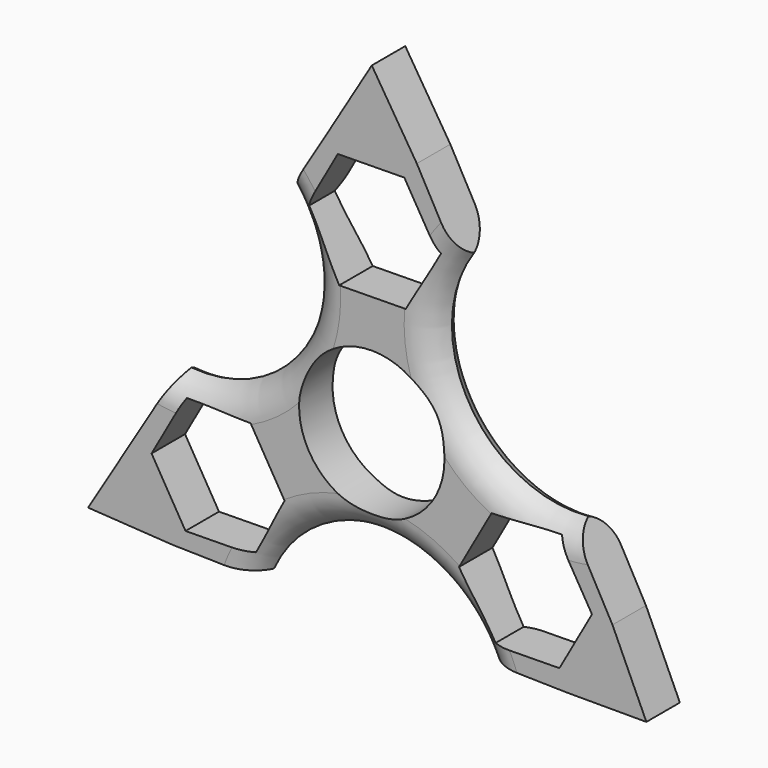
from build123d import *

# Parameters (mm, degrees)
F0_R        = 11.0236
F1_DEPTH    = 6.35
F3_DEPTH    = 6.351
F4_T2_ANGLE = 208.5230453718
F4_T4_ANGLE = 208.5230453718
F5_T2_ANGLE = 208.2569574015
F5_T4_ANGLE = 208.2569574015
F5_T6_ANGLE = 208.3391735822
F5_T8_ANGLE = 208.3391735822


# Not quite as in the source:
# - a fillet or chamfer that OpenCascade refuses, or shapes differently, is made with other operations: its cross-section is extruded or revolved along the edge and cut away or added


with BuildPart() as f1:
    # F0 (on Front) → F1 (new body)
    with BuildSketch(Plane.XZ):
        with BuildLine():
            ThreePointArc((-6.361134185, 38.4869140134), (-13.0376894815, 34.8143114794), (-13.1954000372, 27.1959437158))
            Line((-13.1954000372, 27.1959437158), (-6.361134185, 38.4869140134))
        make_face()
        with BuildLine():
            ThreePointArc((-13.1954000372, 27.1959437158), (-12.0854365863, 25.4236919745), (-11.182896614, 23.5373418757))
            Line((-11.182896614, 23.5373418757), (-6.8342658522, 15.6318107228))
            Line((-6.8342658522, 15.6318107228), (6.361134185, 15.3586480274))
            Line((6.361134185, 15.3586480274), (12.166239176, 24.9493296669))
            ThreePointArc((12.166239176, 24.9493296669), (12.6579537914, 25.813314353), (13.1954000372, 26.649618325))
            Line((13.1954000372, 26.649618325), (6.8342658522, 38.213751318))
            Line((6.8342658522, 38.213751318), (-6.361134185, 38.4869140134))
            Line((-6.361134185, 38.4869140134), (-13.1954000372, 27.1959437158))
        make_face()
        Polygon((-5.1509550469, 35.5981407892), (4.9376044233, 35.7213188292), (10.0885594702, 27.0459590603), (5.1509550469, 18.2474212516), (-4.9376044233, 18.1242432116), (-10.0885594702, 26.7996029805), align=None, mode=Mode.SUBTRACT)
        Polygon((0, 49.0980930626), (-6.361134185, 38.4869140134), (6.8342658522, 38.213751318), align=None)
        with BuildLine():
            ThreePointArc((13.1954000372, 26.649618325), (13.3531105929, 34.2679860885), (6.8342658522, 38.213751318))
            Line((6.8342658522, 38.213751318), (13.1954000372, 26.649618325))
        make_face()
        with BuildLine():
            ThreePointArc((-12.0743322028, 7.6382693135), (3.9762189893, 13.7230586532), (14.2875, 0))
            ThreePointArc((14.2875, 0), (10.1308119649, -10.0746863565), (0.0793732905, -14.2872795217))
            ThreePointArc((0.0793732905, -14.2872795217), (8.9083466238, -16.6700675471), (15.5142475213, -22.9938735391))
            Line((15.5142475213, -22.9938735391), (10.120412267, -13.1882278148))
            Line((10.120412267, -13.1882278148), (16.9546781192, -1.8972575172))
            Line((16.9546781192, -1.8972575172), (26.036317183, -2.0852597754))
            ThreePointArc((26.036317183, -2.0852597754), (12.024896146, 7.8015018829), (12.166239176, 24.9493296669))
            Line((12.166239176, 24.9493296669), (6.361134185, 15.3586480274))
            Line((6.361134185, 15.3586480274), (-6.8342658522, 15.6318107228))
            Line((-6.8342658522, 15.6318107228), (-11.182896614, 23.5373418757))
            ThreePointArc((-11.182896614, 23.5373418757), (-9.8273821058, 15.4868133781), (-12.0743322028, 7.6382693135))
        make_face()
        with BuildLine():
            ThreePointArc((-0.2295262012, -14.2856562318), (-12.3235568651, -7.229287824), (-12.5815056316, 6.7704041454))
            ThreePointArc((-12.5815056316, 6.7704041454), (-19.015460222, 0.5347397877), (-27.6268738812, -1.9396968034))
            Line((-27.6268738812, -1.9396968034), (-16.481546452, -2.1704202126))
            Line((-16.481546452, -2.1704202126), (-10.120412267, -13.7345532056))
            Line((-10.120412267, -13.7345532056), (-14.8142929381, -21.48936819))
            ThreePointArc((-14.8142929381, -21.48936819), (-8.3570392335, -16.196693448), (-0.2295262012, -14.2856562318))
        make_face()
        with BuildLine():
            Line((-16.481546452, -2.1704202126), (-27.6268738812, -1.9396968034))
            ThreePointArc((-27.6268738812, -1.9396968034), (-28.6524995261, -1.9469458697), (-29.6769464892, -1.8972575172))
            Line((-29.6769464892, -1.8972575172), (-36.5112123414, -13.1882278148))
            Line((-36.5112123414, -13.1882278148), (-30.1500781564, -24.7523608078))
            Line((-30.1500781564, -24.7523608078), (-16.9546781192, -25.0255235032))
            ThreePointArc((-16.9546781192, -25.0255235032), (-15.9836520099, -23.1974217673), (-14.8142929381, -21.48936819))
            Line((-14.8142929381, -21.48936819), (-10.120412267, -13.7345532056))
            Line((-10.120412267, -13.7345532056), (-16.481546452, -2.1704202126))
        make_face()
        Polygon((-13.227252834, -13.3382124703), (-18.1648572573, -22.136750279), (-28.2534167275, -22.259928319), (-33.4043717744, -13.5845685501), (-28.4667673511, -4.7860307414), (-18.3782078809, -4.6628527014), align=None, mode=Mode.SUBTRACT)
        with BuildLine():
            Line((-36.5112123414, -13.1882278148), (-29.6769464892, -1.8972575172))
            ThreePointArc((-29.6769464892, -1.8972575172), (-36.3535017857, -5.5698600512), (-36.5112123414, -13.1882278148))
        make_face()
        Polygon((-30.1500781564, -24.7523608078), (-36.5112123414, -13.1882278148), (-43.0257582463, -23.9509850598), align=None)
        with BuildLine():
            ThreePointArc((-30.1500781564, -24.7523608078), (-23.6312334156, -28.6981260373), (-16.9546781192, -25.0255235032))
            Line((-16.9546781192, -25.0255235032), (-30.1500781564, -24.7523608078))
        make_face()
        with BuildLine():
            Line((29.6769464892, -25.0255235032), (16.481546452, -24.7523608078))
            ThreePointArc((16.481546452, -24.7523608078), (23.0003911927, -28.6981260373), (29.6769464892, -25.0255235032))
        make_face()
        Polygon((36.5112123414, -13.7345532056), (29.6769464892, -25.0255235032), (41.6538193822, -25.0255235032), align=None)
        with BuildLine():
            Line((10.120412267, -13.1882278148), (15.5142475213, -22.9938735391))
            ThreePointArc((15.5142475213, -22.9938735391), (16.0217836371, -23.8599777372), (16.481546452, -24.7523608078))
            Line((16.481546452, -24.7523608078), (29.6769464892, -25.0255235032))
            Line((29.6769464892, -25.0255235032), (36.5112123414, -13.7345532056))
            Line((36.5112123414, -13.7345532056), (30.1500781564, -2.1704202126))
            ThreePointArc((30.1500781564, -2.1704202126), (28.0908210273, -2.2426461076), (26.036317183, -2.0852597754))
            Line((26.036317183, -2.0852597754), (16.9546781192, -1.8972575172))
            Line((16.9546781192, -1.8972575172), (10.120412267, -13.1882278148))
        make_face()
        Polygon((18.1648572573, -4.7860307414), (28.2534167275, -4.6628527014), (33.4043717744, -13.3382124703), (28.4667673511, -22.136750279), (18.3782078809, -22.259928319), (13.227252834, -13.5845685501), align=None, mode=Mode.SUBTRACT)
        with BuildLine():
            Line((30.1500781564, -2.1704202126), (36.5112123414, -13.7345532056))
            ThreePointArc((36.5112123414, -13.7345532056), (36.6689228971, -6.1161854421), (30.1500781564, -2.1704202126))
        make_face()
        with BuildLine():
            ThreePointArc((0.0793732905, -14.2872795217), (10.1308119649, -10.0746863565), (14.2875, 0))
            ThreePointArc((14.2875, 0), (3.9762189893, 13.7230586532), (-12.0743322028, 7.6382693135))
            ThreePointArc((-12.0743322028, 7.6382693135), (-12.3220144066, 7.2008861809), (-12.5815056316, 6.7704041454))
            ThreePointArc((-12.5815056316, 6.7704041454), (-12.3235568651, -7.229287824), (-0.2295262012, -14.2856562318))
            ThreePointArc((-0.2295262012, -14.2856562318), (-0.0750730639, -14.2858225171), (0.0793732905, -14.2872795217))
        make_face()
        Circle(F0_R, mode=Mode.SUBTRACT)
    extrude(amount=F1_DEPTH)

    # F2 (on face) → F3 (cut, through all)
    with BuildSketch(Plane.XZ.offset(6.35)):
        with BuildLine():
            Line((-16.9546781192, -25.0255235032), (-30.1500781564, -24.7523608078))
            ThreePointArc((-30.1500781564, -24.7523608078), (-23.6312334156, -28.6981260373), (-16.9546781192, -25.0255235032))
        make_face()
        with BuildLine():
            ThreePointArc((-29.6769464892, -1.8972575172), (-36.3535017857, -5.5698600512), (-36.5112123414, -13.1882278148))
            Line((-36.5112123414, -13.1882278148), (-29.6769464892, -1.8972575172))
        make_face()
        with BuildLine():
            Line((30.1500781564, -2.1704202126), (36.5112123414, -13.7345532056))
            ThreePointArc((36.5112123414, -13.7345532056), (36.6689228971, -6.1161854421), (30.1500781564, -2.1704202126))
        make_face()
        with BuildLine():
            Line((29.6769464892, -25.0255235032), (16.481546452, -24.7523608078))
            ThreePointArc((16.481546452, -24.7523608078), (23.0003911927, -28.6981260373), (29.6769464892, -25.0255235032))
        make_face()
        with BuildLine():
            Line((6.8342658522, 38.213751318), (13.1954000372, 26.649618325))
            ThreePointArc((13.1954000372, 26.649618325), (13.3531105929, 34.2679860885), (6.8342658522, 38.213751318))
        make_face()
        with BuildLine():
            ThreePointArc((-6.361134185, 38.4869140134), (-13.0376894815, 34.8143114794), (-13.1954000372, 27.1959437158))
            Line((-13.1954000372, 27.1959437158), (-6.361134185, 38.4869140134))
        make_face()
    extrude(amount=-F3_DEPTH, mode=Mode.SUBTRACT)

    # F4: fillet of radius 5.08 on 2 edges, made by hand

    # F4_s1 → F4_t2 (revolve, cut)
    with BuildSketch(Plane(origin=(-30.5067493173, 0, 8.3287650763), x_dir=(0, 1, 0), z_dir=(-0.9646936088, 0, 0.263374716))):
        with BuildLine():
            ThreePointArc((-6.35, -32.0437011532), (-4.8621024484, -28.4515987048), (-1.27, -26.9637011532))
            Line((-1.27, -26.9637011532), (-6.35, -26.9637011532))
            Line((-6.35, -26.9637011532), (-6.35, -32.0437011532))
        make_face()
    revolve(axis=Axis((-28.2701906199, -6.35, 16.5208721764), (0, 1, 0)), revolution_arc=F4_T2_ANGLE, mode=Mode.SUBTRACT)

    # F4_s3 → F4_t4 (revolve, cut)
    with BuildSketch(Plane(origin=(-30.5067493173, 0, 8.3287650763), x_dir=(0, 1, 0), z_dir=(-0.9646936088, 0, 0.263374716))):
        with BuildLine():
            ThreePointArc((-5.08, -26.9637011532), (-1.4878975516, -28.4515987048), (0, -32.0437011532))
            Line((0, -32.0437011532), (0, -26.9637011532))
            Line((0, -26.9637011532), (-5.08, -26.9637011532))
        make_face()
    revolve(axis=Axis((-28.2701906199, 0, 16.5208721764), (0, 1, 0)), revolution_arc=F4_T4_ANGLE, mode=Mode.SUBTRACT)

    # F5: fillet of radius 5.08 on 4 edges, made by hand

    # F5_s1 → F5_t2 (revolve, cut)
    with BuildSketch(Plane(origin=(22.5566144239, 0, 22.2411685485), x_dir=(0, 1, 0), z_dir=(0.7120682565, 0, 0.7021102464))):
        with BuildLine():
            ThreePointArc((-6.35, -31.9942361937), (-4.8621024484, -28.4021337453), (-1.27, -26.9142361937))
            Line((-1.27, -26.9142361937), (-6.35, -26.9142361937))
            Line((-6.35, -26.9142361937), (-6.35, -31.9942361937))
        make_face()
    revolve(axis=Axis((28.4734455715, -6.35, 16.2404191492), (0, 1, 0)), revolution_arc=F5_T2_ANGLE, mode=Mode.SUBTRACT)

    # F5_s3 → F5_t4 (revolve, cut)
    with BuildSketch(Plane(origin=(22.5566144239, 0, 22.2411685485), x_dir=(0, 1, 0), z_dir=(0.7120682565, 0, 0.7021102464))):
        with BuildLine():
            ThreePointArc((0, -31.9942361937), (-1.4878975516, -28.4021337453), (-5.08, -26.9142361937))
            Line((-5.08, -26.9142361937), (0, -26.9142361937))
            Line((0, -26.9142361937), (0, -31.9942361937))
        make_face()
    revolve(axis=Axis((28.4734455715, 0, 16.2404191492), (0, 1, 0)), revolution_arc=F5_T4_ANGLE, mode=Mode.SUBTRACT)

    # F5_s5 → F5_t6 (revolve, cut)
    with BuildSketch(Plane(origin=(8.0008610832, 0, -30.6332127592), x_dir=(0, 1, 0), z_dir=(0.2527054311, 0, -0.9675432626))):
        with BuildLine():
            ThreePointArc((0, -32.0095340444), (-1.4878975516, -28.417431596), (-5.08, -26.9295340444))
            Line((-5.08, -26.9295340444), (0, -26.9295340444))
            Line((0, -26.9295340444), (0, -32.0095340444))
        make_face()
    revolve(axis=Axis((-0.1721976202, 0, -32.7678731954), (0, 1, 0)), revolution_arc=F5_T6_ANGLE, mode=Mode.SUBTRACT)

    # F5_s7 → F5_t8 (revolve, cut)
    with BuildSketch(Plane(origin=(8.0008610832, 0, -30.6332127592), x_dir=(0, 1, 0), z_dir=(0.2527054311, 0, -0.9675432626))):
        with BuildLine():
            ThreePointArc((-6.35, -32.0095340444), (-4.8621024484, -28.417431596), (-1.27, -26.9295340444))
            Line((-1.27, -26.9295340444), (-6.35, -26.9295340444))
            Line((-6.35, -26.9295340444), (-6.35, -32.0095340444))
        make_face()
    revolve(axis=Axis((-0.1721976202, -6.35, -32.7678731954), (0, 1, 0)), revolution_arc=F5_T8_ANGLE, mode=Mode.SUBTRACT)


solid = f1.part
